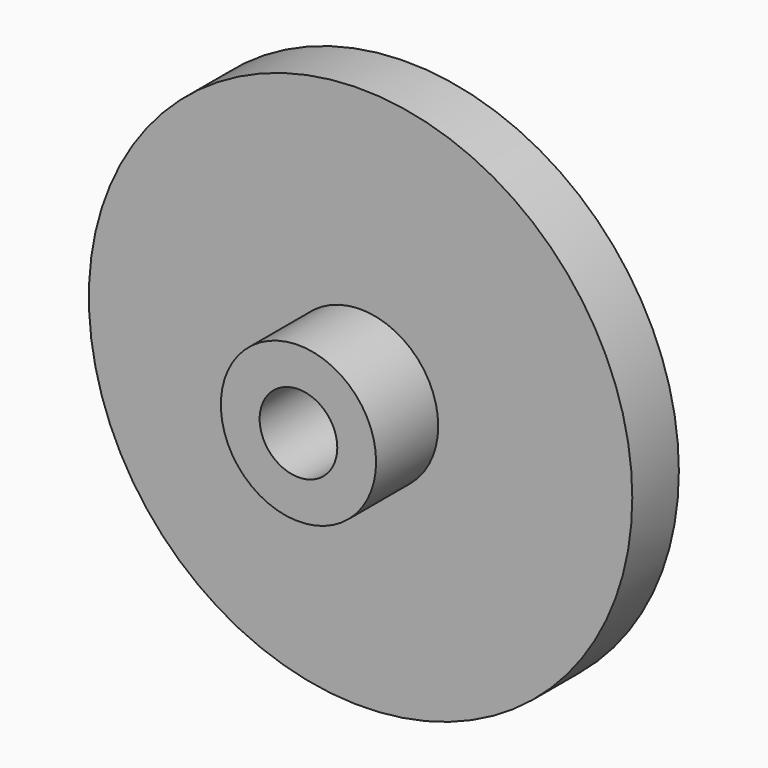
from build123d import *

# Parameters (mm, degrees)
F0_R          = 22.225
F1_DEPTH      = 4.7625
F2_R          = 6.35
F3_DEPTH      = 6.35
F4_R          = 3.175
F5_DEPTH      = 25.4
F5_DEPTH_BACK = 73


# Not quite as in the source:
# - an extrude ends at something that could not be found from the text; its depth is read off the source's solid


with BuildPart() as f1:
    # F0 (on Front) → F1 (new body)
    with BuildSketch(Plane.XZ):
        Circle(F0_R)
    extrude(amount=F1_DEPTH)

    # F2 (on face) → F3 (join)
    with BuildSketch(Plane.XZ.offset(4.7625)):
        Circle(F2_R)
    extrude(amount=F3_DEPTH)

    # F4 (on face) → F5 (cut, two sides)
    with BuildSketch(Plane.XZ.offset(11.1125)) as f5_sk:
        Circle(F4_R)
    extrude(amount=-F5_DEPTH, mode=Mode.SUBTRACT)
    extrude(f5_sk.sketch, amount=F5_DEPTH_BACK, mode=Mode.SUBTRACT)


solid = f1.part
